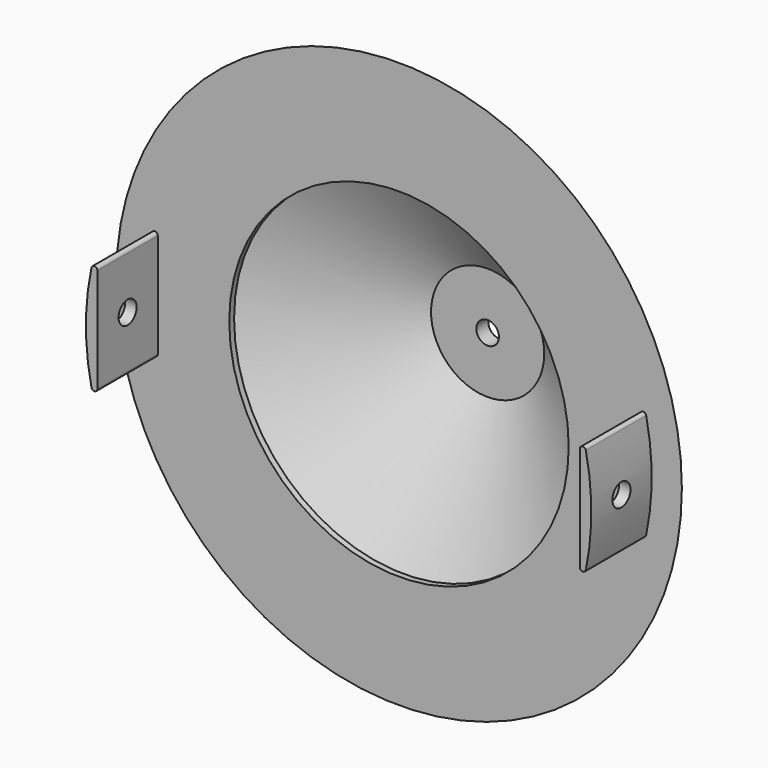
from build123d import *

# Parameters (mm, degrees)
F3_DEPTH = 10
F4_R     = 1.5
F5_DEPTH = 25
F6_R     = 1.5
F7_DEPTH = 25
F8_F1_R  = 0.4
F8_F2_R  = 0.4
F8_F3_R  = 0.4
F8_F4_R  = 0.4


# Not quite as in the source:
# - a feature names something its author has since deleted; it is built from what else it names


with BuildPart() as f1:
    # F0 (on Top) → F1 (revolve)
    with BuildSketch(Plane.XY):
        Polygon((22.5, 0.8), (22.5, 0), (37.5, 0), (7.5, 16.6666666667), (1.5, 16.6666666667), (1.5, 14.6888888889), (7.5, 14.6888888889), (32.5, 0.8), align=None)
    revolve(axis=Axis((0, 10, 0), (0, 1, 0)))

    # F2 (on face) → F3 (join)
    with BuildSketch(Plane.XZ):
        with BuildLine():
            Line((-31.9726445575, -10), (-31.9726445575, 10))
            ThreePointArc((-31.9726445575, 10), (-33.5, 0), (-31.9726445575, -10))
        make_face()
        with BuildLine():
            ThreePointArc((31.9726445575, -10), (33.5, 0), (31.9726445575, 10))
            Line((31.9726445575, 10), (31.9726445575, -10))
        make_face()
    extrude(amount=F3_DEPTH)

    # F4 (on face) → F5 (cut)
    with BuildSketch(Plane.YZ.offset(-31.9726445575)):
        with Locations((-5, 0)):
            Circle(F4_R)
    extrude(amount=-F5_DEPTH, mode=Mode.SUBTRACT)

    # F6 (on face) → F7 (cut)
    with BuildSketch(Plane(origin=(31.9726445575, 0, 0), x_dir=(0, -1, 0), z_dir=(-1, 0, 0))):
        with Locations((5, 0)):
            Circle(F6_R)
    extrude(amount=-F7_DEPTH, mode=Mode.SUBTRACT)

    # F8: fillet of radius 0.4 on 4 edges, made by hand

    # F8_f1
    f8_f1_edges = [f1.edges().sort_by_distance(p)[0] for p in [
        (31.9726445575, -5, 10),
    ]]
    fillet(f8_f1_edges, radius=F8_F1_R)

    # F8_f2
    f8_f2_edges = [f1.edges().sort_by_distance(p)[0] for p in [
        (31.9726445575, -5, -10),
    ]]
    fillet(f8_f2_edges, radius=F8_F2_R)

    # F8_f3
    f8_f3_edges = [f1.edges().sort_by_distance(p)[0] for p in [
        (-31.9726445575, -5, -10),
    ]]
    fillet(f8_f3_edges, radius=F8_F3_R)

    # F8_f4
    f8_f4_edges = [f1.edges().sort_by_distance(p)[0] for p in [
        (-31.9726445575, -5, 10),
    ]]
    fillet(f8_f4_edges, radius=F8_F4_R)


solid = f1.part
